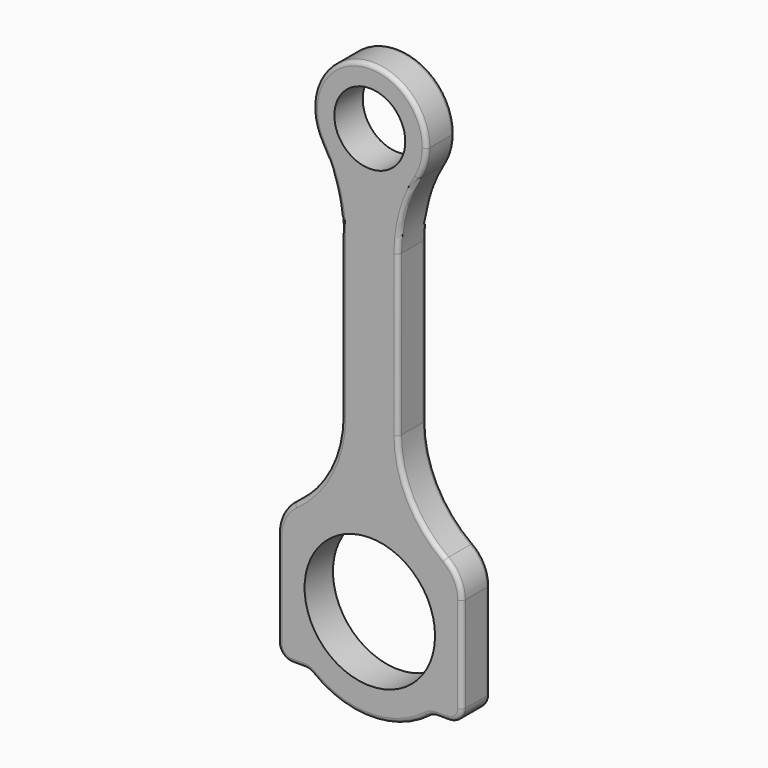
from build123d import *

# Parameters (mm, degrees)
F0_R     = 4.6
F0_R_2   = 2.5
F1_DEPTH = 2.5
F3_DEPTH = 1.3
F4_R     = 1
F6_R     = 0.5
F7_R     = 0.3


# Not quite as in the source:
# - two fillets or chamfers of one size are made in one step


with BuildPart() as f1:
    # F0 (on Front) → F1 (new body)
    with BuildSketch(Plane.XZ):
        with BuildLine():
            Line((-6.5, -5), (-4.3081318457, -5))
            ThreePointArc((-4.3081318457, -5), (0, -6.6), (4.3081318457, -5))
            Line((4.3081318457, -5), (6.5, -5))
            Line((6.5, -5), (6.5, 2.7331300737))
            ThreePointArc((6.5, 2.7331300737), (6.1913182588, 4.0111493746), (5.3333333333, 5.0073820875))
            ThreePointArc((5.3333333333, 5.0073820875), (2.881947832, 7.8537612674), (2, 11.5052449841))
            Line((2, 11.5052449841), (2, 22.7888974491))
            ThreePointArc((2, 22.7888974491), (2.3637588834, 25.4615098682), (3.4285714286, 27.9396849854))
            ThreePointArc((3.4285714286, 27.9396849854), (0, 26), (-3.4285714286, 27.9396849854))
            ThreePointArc((-3.4285714286, 27.9396849854), (-2.3637588834, 25.4615098682), (-2, 22.7888974491))
            Line((-2, 22.7888974491), (-2, 11.5052449841))
            ThreePointArc((-2, 11.5052449841), (-2.881947832, 7.8537612674), (-5.3333333333, 5.0073820875))
            ThreePointArc((-5.3333333333, 5.0073820875), (-6.1913182588, 4.0111493746), (-6.5, 2.7331300737))
            Line((-6.5, 2.7331300737), (-6.5, -5))
        make_face()
        Circle(F0_R, mode=Mode.SUBTRACT)
        with BuildLine():
            ThreePointArc((4, 30), (-1.0690449676, 33.8544964466), (-3.4285714286, 27.9396849854))
            ThreePointArc((-3.4285714286, 27.9396849854), (0, 26), (3.4285714286, 27.9396849854))
            ThreePointArc((3.4285714286, 27.9396849854), (3.8544964466, 28.9309550324), (4, 30))
        make_face()
        with Locations((0, 30)):
            Circle(F0_R_2, mode=Mode.SUBTRACT)
    extrude(amount=F1_DEPTH)

    # F2 (on face) → F3 (cut)
    with BuildSketch(Plane(origin=(0, 0, 0), x_dir=(-1, 0, 0), z_dir=(0, 1, 0))):
        with BuildLine():
            Line((1.25, 26), (-1.25, 26))
            Line((-1.25, 26), (-1.25, 10))
            ThreePointArc((-1.25, 10), (-1.5963426761, 7.9065574908), (-2.5984620121, 6.0362068218))
            ThreePointArc((-2.5984620121, 6.0362068218), (-2.614191014, 5.3258360734), (-1.9409695348, 5.098576659))
            ThreePointArc((-1.9409695348, 5.098576659), (-0.9821174529, 5.3241952301), (0, 5.4))
            ThreePointArc((0, 5.4), (0.9821174529, 5.3241952301), (1.9409695348, 5.098576659))
            ThreePointArc((1.9409695348, 5.098576659), (2.614191014, 5.3258360734), (2.5984620121, 6.0362068218))
            ThreePointArc((2.5984620121, 6.0362068218), (1.5963426761, 7.9065574908), (1.25, 10))
            Line((1.25, 10), (1.25, 26))
        make_face()
    extrude(amount=-F3_DEPTH, mode=Mode.SUBTRACT)

    # F4
    f4_edges = [f1.edges().sort_by_distance(p)[0] for p in [
        (1.25, -0.65, 26),
        (-1.25, -0.65, 26),
        (-6.5, -1.25, -5),
        (-4.308132, -1.25, -5),
        (6.5, -1.25, -5),
        (4.308132, -1.25, -5),
    ]]
    fillet(f4_edges, radius=F4_R)

    # F6
    f6_edges = [f1.edges().sort_by_distance(p)[0] for p in [
        (0, -1.3, 5.4),
        (1.25, -1.3, 17.5),
        (0.957107, -1.3, 25.707107),
        (1.596343, -1.3, 7.906557),
        (0, -1.3, 26),
        (2.614191, -1.3, 5.325836),
        (-0.957107, -1.3, 25.707107),
        (-1.25, -1.3, 17.5),
        (-2.614191, -1.3, 5.325836),
        (-1.596343, -1.3, 7.906557),
    ]]
    fillet(f6_edges, radius=F6_R)

    # F7
    f7_edges = [f1.edges().sort_by_distance(p)[0] for p in [
        (2.614191, 0, 5.325836),
        (6.5, 0, -0.633435),
        (2.881948, -2.5, 7.853761),
        (1.25, 0, 17.5),
        (0.957107, 0, 25.707107),
        (-6.5, 0, -0.633435),
        (-6.207107, 0, -4.707107),
        (-6.191318, 0, 4.011149),
        (-5.082381, 0, -5),
        (-2.881948, 0, 7.853761),
        (-4.340319, 0, -5.054095),
        (-2, 0, 17.147071),
        (0, 0, -6.6),
        (-2.363759, 0, 25.46151),
        (4.340319, 0, -5.054095),
        (0, 0, 34),
        (5.082381, 0, -5),
        (2.363759, 0, 25.46151),
        (6.207107, 0, -4.707107),
        (2, 0, 17.147071),
        (2.881948, 0, 7.853761),
        (6.191318, 0, 4.011149),
        (1.596343, 0, 7.906557),
        (0, 0, 26),
        (-0.957107, 0, 25.707107),
        (0, 0, 5.4),
        (-1.25, 0, 17.5),
        (-2.614191, 0, 5.325836),
        (-1.596343, 0, 7.906557),
        (-6.5, -2.5, -0.633435),
        (-6.207107, -2.5, -4.707107),
        (-6.191318, -2.5, 4.011149),
        (-5.082381, -2.5, -5),
        (-2.881948, -2.5, 7.853761),
        (-4.340319, -2.5, -5.054095),
        (-2, -2.5, 17.147071),
        (0, -2.5, -6.6),
        (-2.363759, -2.5, 25.46151),
        (4.340319, -2.5, -5.054095),
        (0, -2.5, 34),
        (5.082381, -2.5, -5),
        (2.363759, -2.5, 25.46151),
        (6.207107, -2.5, -4.707107),
        (2, -2.5, 17.147071),
        (6.5, -2.5, -0.633435),
        (6.191318, -2.5, 4.011149),
    ]]
    fillet(f7_edges, radius=F7_R)


solid = f1.part
